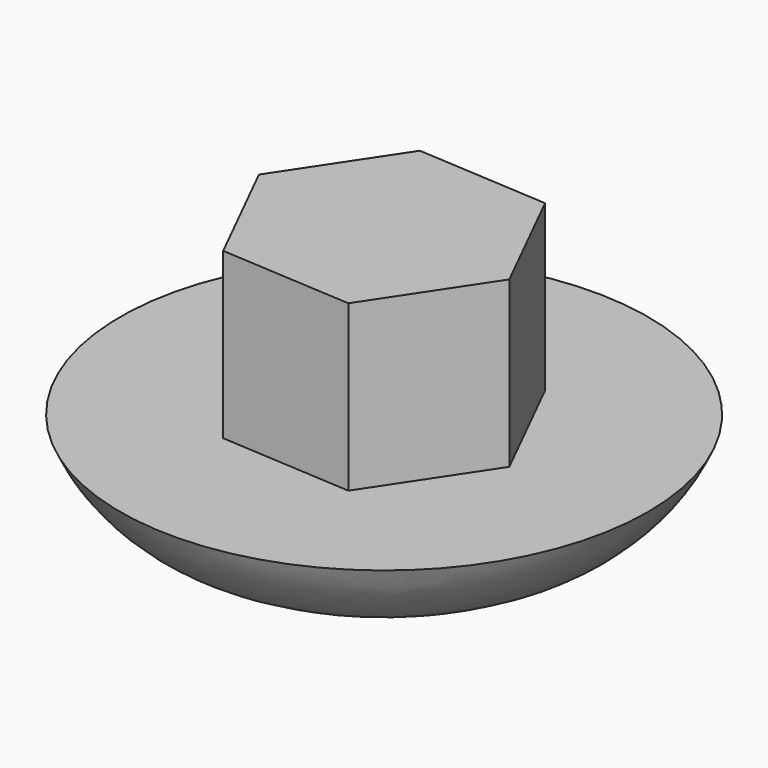
from build123d import *

# Parameters (mm, degrees)
F1_DEPTH = 5
F2_R     = 8
F3_DEPTH = 3


# Not quite as in the source:
# - a fillet or chamfer that OpenCascade refuses, or shapes differently, is made with other operations: its cross-section is extruded or revolved along the edge and cut away or added


with BuildPart() as f1:
    # F0 (on Top) → F1 (new body)
    with BuildSketch(Plane.XY):
        Polygon((4.5920703038, -0.2481590048), (2.8108349475, 3.333349142), (-1.1814597696, 3.5815081468), (-3.3925191305, 0.2481590048), (-1.6112837742, -3.333349142), (2.3810109429, -3.5815081468), align=None)
    extrude(amount=F1_DEPTH)

    # F2 (on face) → F3 (join)
    with BuildSketch(Plane(origin=(0, 0, 0), x_dir=(1, 0, 0), z_dir=(0, 0, -1))):
        with Locations((0.5997755867, 0)):
            Circle(F2_R)
        Polygon((2.8108349475, -3.333349142), (-1.1814597696, -3.5815081468), (-3.3925191305, -0.2481590048), (-1.6112837742, 3.333349142), (2.3810109429, 3.5815081468), (4.5920703038, 0.2481590048), align=None, mode=Mode.SUBTRACT)
        Polygon((-3.3925191305, -0.2481590048), (-1.1814597696, -3.5815081468), (2.8108349475, -3.333349142), (4.5920703038, 0.2481590048), (2.3810109429, 3.5815081468), (-1.6112837742, 3.333349142), align=None)
    extrude(amount=F3_DEPTH)

    # F4: fillet of radius 5 on 1 edges, made by hand

    # F4_s1 → F4_t2 (revolve, cut)
    with BuildSketch(Plane.XZ):
        with BuildLine():
            ThreePointArc((8.5997755867, 0), (6.7558126792, -2.1833001327), (4.0171998917, -3))
            Line((4.0171998917, -3), (8.5997755867, -3))
            Line((8.5997755867, -3), (8.5997755867, 0))
        make_face()
    revolve(axis=Axis((0.5997755867, 0, -3), (0, 0, -1)), mode=Mode.SUBTRACT)


solid = f1.part
